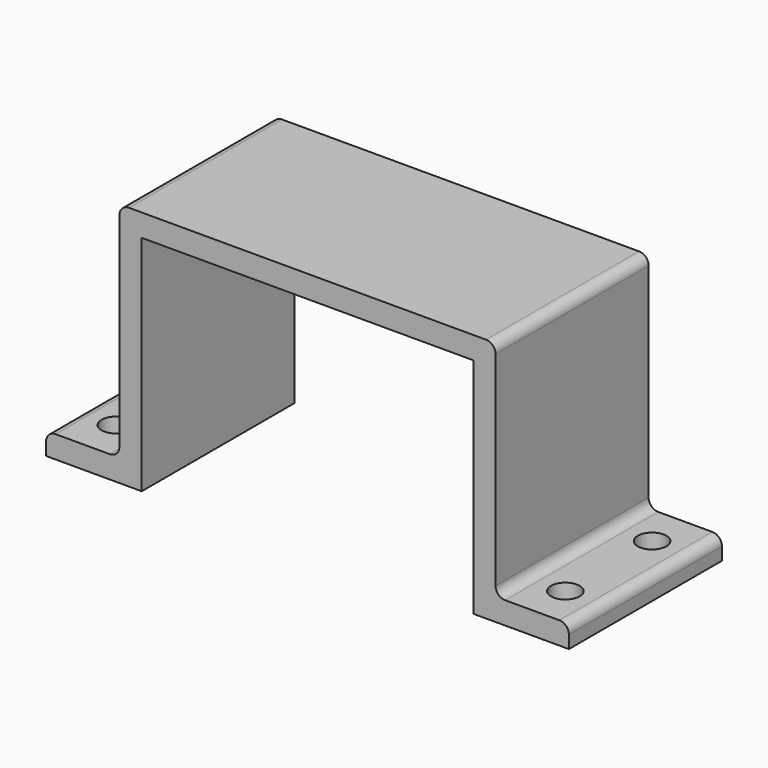
from build123d import *

# Parameters (mm, degrees)
F1_DEPTH = 30
F2_R     = 2.2479
F3_DEPTH = 3.5
F4_R     = 1.5


# Not quite as in the source:
# - a pattern or mirror of a feature is missing from the dataset's text; its kind, count and spacing are read off the source's solid


with BuildPart() as f1:
    # F0 (on Front) → F1 (new body)
    with BuildSketch(Plane.XZ):
        Polygon((-26, 0), (-26, 31.5), (26, 31.5), (26, 0), (29.5, 0), (29.5, 35), (-29.5, 35), (-29.5, 0), align=None)
        Polygon((-26, -3.5), (-26, 0), (-29.5, 0), (-41, 0), (-41, -3.5), align=None)
        Polygon((29.5, 0), (26, 0), (26, -3.5), (41, -3.5), (41, 0), align=None)
    extrude(amount=F1_DEPTH)

    # F2 (on face) → F3 (cut, through all)
    with BuildSketch(Plane.XY):
        with Locations((-35.25, -23.5)):
            Circle(F2_R)
        with Locations((-35.25, -6.5)):
            Circle(F2_R)
    f3 = extrude(amount=-F3_DEPTH, mode=Mode.SUBTRACT)

    # F3_copies: F3 across plane
    add(f3.mirror(Plane(origin=(0, 0, 0), x_dir=(0, 0, 1), z_dir=(1, 0, 0))), mode=Mode.SUBTRACT)

    # F4
    f4_edges = [f1.edges().sort_by_distance(p)[0] for p in [
        (-29.5, -15, 35),
        (-29.5, -15, 0),
        (-41, -15, 0),
        (29.5, -15, 35),
        (29.5, -15, 0),
        (41, -15, 0),
    ]]
    fillet(f4_edges, radius=F4_R)


solid = f1.part
